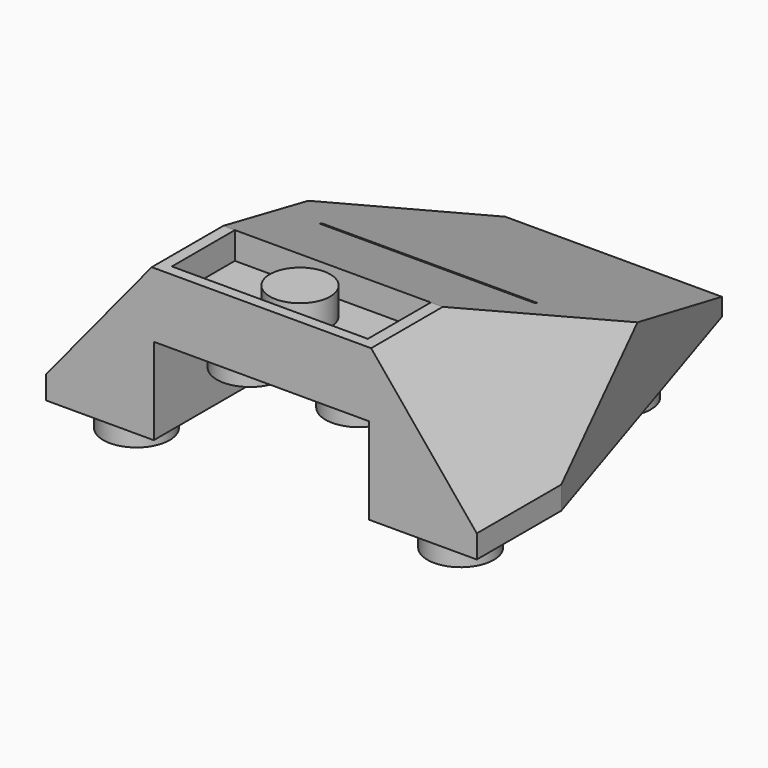
from build123d import *

# Parameters (mm, degrees)
F0_W      = 15.96
F0_H      = 8.3576925244
F1_DEPTH  = 32.5
F2_W      = 15.9
F2_H      = 6.4
F3_DEPTH  = 15.5
F4_DEPTH  = 70
F6_DEPTH  = 25
F7_R      = 2.45
F8_DEPTH  = 2
F7_W      = 15.9
F7_H      = 7.8
F8_FACE_R = 2.45
F9_DEPTH  = 1.5
F10_R     = 2.45
F10_R_2   = 1.55
F11_DEPTH = 5.9
F12_R     = 2.45
F12_R_2   = 1.55
F13_DEPTH = 1.9
F14_DEPTH = 4
F15_DEPTH = 4
F16_W     = 14.4657706842
F16_H     = 5.8139935136
F16_R     = 2.228006958
F17_DEPTH = 2
F19_DEPTH = 12.5


with BuildPart() as f1:
    # F0 (on Front) → F1 (new body)
    with BuildSketch(Plane.XZ):
        Polygon((15.9, 3.1903535793), (-15.9, 3.1903535793), (-15.9, -6.5096464207), (-6.726923441, -6.5096464207), (-6.726923441, 1.8480461037), (9.233076559, 1.8480461037), (9.233076559, -6.5096464207), (15.9, -6.5096464207), align=None)
        with Locations((1.253076559, -2.3308001585)):
            Rectangle(F0_W, F0_H)
    extrude(amount=F1_DEPTH)

    # F2 (on face) → F3 (cut)
    with BuildSketch(Plane.XZ.offset(32.5)):
        with Locations((0, -3.3096464207)):
            Rectangle(F2_W, F2_H)
    extrude(amount=-F3_DEPTH, mode=Mode.SUBTRACT)

    # F2 (on face) → F4 (cut)
    with BuildSketch(Plane.XZ.offset(32.5)):
        Polygon((-15.9, 3.1903535793), (-15.9, -6.3096464207), (-8.1, 3.1903535793), align=None)
        Polygon((8.1, 3.1903535793), (15.9, -6.3096464207), (15.9, 3.1903535793), align=None)
    extrude(amount=-F4_DEPTH, mode=Mode.SUBTRACT)

    # F5 (on face) → F6 (cut)
    with BuildSketch(Plane(origin=(0, 0, -6.5096464207), x_dir=(1, 0, 0), z_dir=(0, 0, -1))):
        Polygon((-8, 0), (-15.9, 24.7), (-15.9, 0), align=None)
        Polygon((15.9, 24.7), (8, 0), (15.9, 0), align=None)
    extrude(amount=-F6_DEPTH, mode=Mode.SUBTRACT)

    # F7 (on face) → F8 (join)
    with BuildSketch(Plane(origin=(0, 0, -0.1096464207), x_dir=(1, 0, 0), z_dir=(0, 0, -1))):
        with Locations((-4.0132352151, 28.5375677049)):
            Circle(F7_R)
        with Locations((4.0132352151, 28.5375677049)):
            Circle(F7_R)
    extrude(amount=F8_DEPTH)

    # F7 (on face) + F1_face1 (on face) + F8_face (on face) → F9 (join)
    with BuildSketch(Plane(origin=(0, 0, -0.1096464207), x_dir=(1, 0, 0), z_dir=(0, 0, -1))):
        with Locations((0, 28.6)):
            Rectangle(F7_W, F7_H)
        with Locations((-4.0132352151, 28.5375677049)):
            Circle(F7_R, mode=Mode.SUBTRACT)
        with Locations((4.0132352151, 28.5375677049)):
            Circle(F7_R, mode=Mode.SUBTRACT)
    with BuildSketch(Plane(origin=(0, -13.5883838384, -6.5096464207), x_dir=(1, 0, 0), z_dir=(0, 0, -1))):
        Polygon((-8, -13.5883838384), (8, -13.5883838384), (15.9, 11.1116161616), (15.9, 18.9116161616), (7.95, 18.9116161616), (7.95, 3.4116161616), (-7.95, 3.4116161616), (-7.95, 18.9116161616), (-15.9, 18.9116161616), (-15.9, 11.1116161616), align=None)
    with BuildSketch(Plane(origin=(-4.0132352151, -28.5375677049, -2.1096464207), x_dir=(1, 0, 0), z_dir=(0, 0, -1))):
        Circle(F8_FACE_R)
        with Locations((8.0264704302, 0)):
            Circle(F8_FACE_R)
    extrude(amount=F9_DEPTH)

    # F10 (on face) → F11 (join)
    with BuildSketch(Plane(origin=(0, 0, -0.1096464207), x_dir=(1, 0, 0), z_dir=(0, 0, -1))):
        with Locations((-3.7897760311, 20.9340956062)):
            Circle(F10_R)
        with Locations((-3.7897760311, 20.9340956062)):
            Circle(F10_R_2, mode=Mode.SUBTRACT)
        with Locations((3.8324711446, 20.9340956062)):
            Circle(F10_R)
        with Locations((3.8324711446, 20.9340956062)):
            Circle(F10_R_2, mode=Mode.SUBTRACT)
    extrude(amount=F11_DEPTH)

    # F12 (on face) → F13 (join)
    with BuildSketch(Plane(origin=(0, 0, -8.0096464207), x_dir=(1, 0, 0), z_dir=(0, 0, -1))):
        with Locations((-11.9673879817, 29.0735326707)):
            Circle(F12_R)
        with Locations((-11.9673879817, 29.0735326707)):
            Circle(F12_R_2, mode=Mode.SUBTRACT)
        with Locations((11.9673879817, 29.0735326707)):
            Circle(F12_R)
        with Locations((11.9673879817, 29.0735326707)):
            Circle(F12_R_2, mode=Mode.SUBTRACT)
    extrude(amount=F13_DEPTH)

    # F12 (on face) → F14 (join)
    with BuildSketch(Plane(origin=(0, 0, -8.0096464207), x_dir=(1, 0, 0), z_dir=(0, 0, -1))):
        with Locations((-4.5118764974, 12.756055221)):
            Circle(F12_R)
        with Locations((-4.5118764974, 12.756055221)):
            Circle(F12_R_2, mode=Mode.SUBTRACT)
        with Locations((4.5118764974, 12.756055221)):
            Circle(F12_R)
        with Locations((4.5118764974, 12.756055221)):
            Circle(F12_R_2, mode=Mode.SUBTRACT)
    extrude(amount=F14_DEPTH)

    # F12 (on face) → F15 (join)
    with BuildSketch(Plane(origin=(0, 0, -8.0096464207), x_dir=(1, 0, 0), z_dir=(0, 0, -1))):
        with Locations((-4.7830846161, 5.5871135555)):
            Circle(F12_R)
        with Locations((-4.7830846161, 5.5871135555)):
            Circle(F12_R_2, mode=Mode.SUBTRACT)
        with Locations((4.7830846161, 5.5871135555)):
            Circle(F12_R)
        with Locations((4.7830846161, 5.5871135555)):
            Circle(F12_R_2, mode=Mode.SUBTRACT)
    extrude(amount=F15_DEPTH)

    # F16 (on face) → F17 (cut)
    with BuildSketch(Plane.XY.offset(3.1903535793)):
        with Locations((-0.0129453838, -28.7997983396)):
            Rectangle(F16_W, F16_H)
        with Locations((0, -28.9382264018)):
            Circle(F16_R, mode=Mode.SUBTRACT)
    extrude(amount=-F17_DEPTH, mode=Mode.SUBTRACT)

    # F18 (on Right) → F19 (cut, symmetric)
    with BuildSketch(Plane.YZ):
        Polygon((-25.8897673339, 3.1903535793), (0, -6.7096464207), (0, 3.1903535793), (-0.3126582278, 3.1903535793), align=None)
    extrude(amount=F19_DEPTH, both=True, mode=Mode.SUBTRACT)


solid = f1.part
